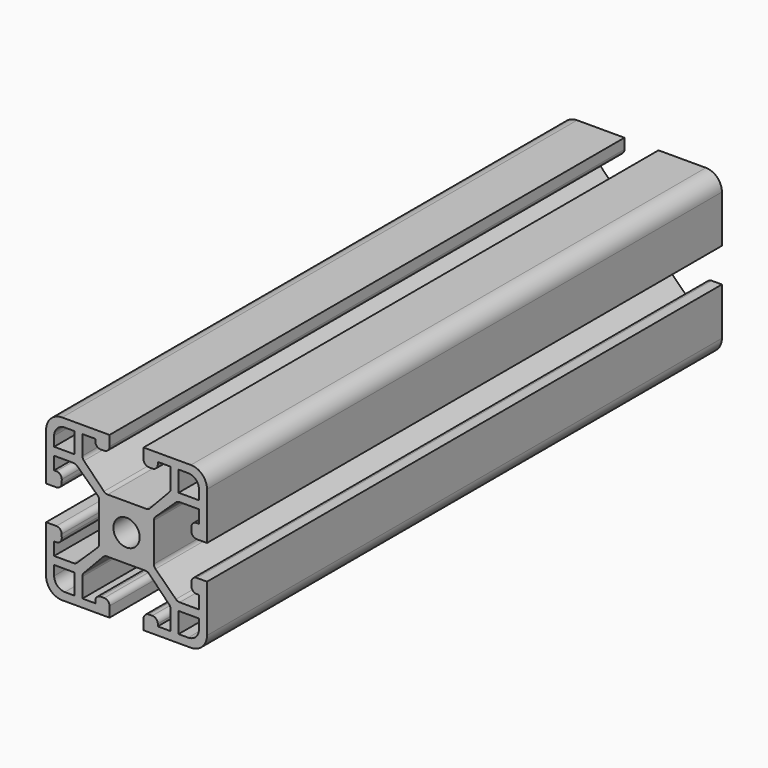
from build123d import *

# Parameters (mm, degrees)
F0_R     = 2.45
F1_DEPTH = 460
F2_DEPTH = 340


# Not quite as in the source:
# - ends of sketch curves that miss each other by under 0.0002 mm in the source are joined


with BuildPart() as f1:
    # F0 (on Front) → F1 (new body)
    with BuildSketch(Plane.XZ):
        with BuildLine():
            Line((-3.1749674082, 15), (-12, 15))
            ThreePointArc((-12, 15), (-14.1213203436, 14.1213203436), (-15, 12))
            Line((-15, 12), (-15, 3.175))
            Line((-15, 3.175), (-13.0855346263, 3.175))
            ThreePointArc((-13.0855346263, 3.175), (-12.3835980145, 3.4627605788), (-12.0856407741, 4.1604300138))
            Line((-12.0856407741, 4.1604300138), (-12.0761692778, 4.8104300138))
            ThreePointArc((-12.0761692778, 4.8104300138), (-12.3638237087, 5.5269366118), (-13.0760631299, 5.825))
            Line((-13.0760631299, 5.825), (-13.5, 5.825))
            Line((-13.5, 5.825), (-13.5, 8.225))
            Line((-13.5, 8.225), (-9.8968845016, 8.225))
            ThreePointArc((-9.8968845016, 8.225), (-9.5279915195, 8.1544718757), (-9.2111331975, 7.9528359354))
            Line((-9.2111331975, 7.9528359354), (-5.4142486959, 4.3754933338))
            ThreePointArc((-5.4142486959, 4.3754933338), (-5.1819174045, 4.0440465354), (-5.1, 3.6476573984))
            Line((-5.1, 3.6476573984), (-5.1, -3.4999243287))
            ThreePointArc((-5.1, -3.4999243287), (-5.1782354607, -3.8876744211), (-5.4007002683, -4.2147528992))
            Line((-5.4007002683, -4.2147528992), (-9.2084959767, -7.9398285705))
            ThreePointArc((-9.2084959767, -7.9398285705), (-9.5301904718, -8.1509666761), (-9.9077957084, -8.225))
            Line((-9.9077957084, -8.225), (-13.5, -8.225))
            Line((-13.5, -8.225), (-13.5, -5.825))
            Line((-13.5, -5.825), (-13.0760631299, -5.825))
            ThreePointArc((-13.0760631299, -5.825), (-12.3638237087, -5.5269366118), (-12.0761692778, -4.8104300138))
            Line((-12.0761692778, -4.8104300138), (-12.0856407741, -4.1604300138))
            ThreePointArc((-12.0856407741, -4.1604300138), (-12.3835980145, -3.4627605788), (-13.0855346263, -3.175))
            Line((-13.0855346263, -3.175), (-15, -3.175))
            Line((-15, -3.175), (-15, -12))
            ThreePointArc((-15, -12), (-14.1213203436, -14.1213203436), (-12, -15))
            Line((-12, -15), (-3.175, -15))
            Line((-3.175, -15), (-3.175, -13.0855346263))
            ThreePointArc((-3.175, -13.0855346263), (-3.4627605788, -12.3835980145), (-4.1604300138, -12.0856407741))
            Line((-4.1604300138, -12.0856407741), (-4.8104300138, -12.0761692778))
            ThreePointArc((-4.8104300138, -12.0761692778), (-5.5269366118, -12.3638237087), (-5.825, -13.0760631299))
            Line((-5.825, -13.0760631299), (-5.825, -13.5))
            Line((-5.825, -13.5), (-8.225, -13.5))
            Line((-8.225, -13.5), (-8.225, -9.8968845016))
            ThreePointArc((-8.225, -9.8968845016), (-8.1544718757, -9.5279915195), (-7.9528359354, -9.2111331975))
            Line((-7.9528359354, -9.2111331975), (-4.3754933338, -5.4142486959))
            ThreePointArc((-4.3754933338, -5.4142486959), (-4.0440465354, -5.1819174045), (-3.6476573984, -5.1))
            Line((-3.6476573984, -5.1), (3.4999243287, -5.1))
            ThreePointArc((3.4999243287, -5.1), (3.8876744211, -5.1782354607), (4.2147528992, -5.4007002683))
            Line((4.2147528992, -5.4007002683), (7.9398285705, -9.2084959767))
            ThreePointArc((7.9398285705, -9.2084959767), (8.1509666761, -9.5301904718), (8.225, -9.9077957084))
            Line((8.225, -9.9077957084), (8.225, -13.5))
            Line((8.225, -13.5), (5.825, -13.5))
            Line((5.825, -13.5), (5.825, -13.0760631299))
            ThreePointArc((5.825, -13.0760631299), (5.5269366118, -12.3638237087), (4.8104300138, -12.0761692778))
            Line((4.8104300138, -12.0761692778), (4.1604300138, -12.0856407741))
            ThreePointArc((4.1604300138, -12.0856407741), (3.4627605788, -12.3835980145), (3.175, -13.0855346263))
            Line((3.175, -13.0855346263), (3.175, -15))
            Line((3.175, -15), (12, -15))
            ThreePointArc((12, -15), (14.1213203436, -14.1213203436), (15, -12))
            Line((15, -12), (15, -3.175))
            Line((15, -3.175), (13.0855346263, -3.175))
            ThreePointArc((13.0855346263, -3.175), (12.3835980145, -3.4627605788), (12.0856407741, -4.1604300138))
            Line((12.0856407741, -4.1604300138), (12.0761692778, -4.8104300138))
            ThreePointArc((12.0761692778, -4.8104300138), (12.3638237087, -5.5269366118), (13.0760631299, -5.825))
            Line((13.0760631299, -5.825), (13.5, -5.825))
            Line((13.5, -5.825), (13.5, -8.225))
            Line((13.5, -8.225), (9.9077957084, -8.225))
            ThreePointArc((9.9077957084, -8.225), (9.5301904718, -8.1509666761), (9.2084959767, -7.9398285705))
            Line((9.2084959767, -7.9398285705), (5.4007002683, -4.2147528992))
            ThreePointArc((5.4007002683, -4.2147528992), (5.1782354607, -3.8876744211), (5.1, -3.4999243287))
            Line((5.1, -3.4999243287), (5.1, 3.6476573984))
            ThreePointArc((5.1, 3.6476573984), (5.1819174045, 4.0440465354), (5.4142486959, 4.3754933338))
            Line((5.4142486959, 4.3754933338), (9.2111331975, 7.9528359354))
            ThreePointArc((9.2111331975, 7.9528359354), (9.5279915195, 8.1544718757), (9.8968845016, 8.225))
            Line((9.8968845016, 8.225), (13.5, 8.225))
            Line((13.5, 8.225), (13.5, 5.825))
            Line((13.5, 5.825), (13.0760631299, 5.825))
            ThreePointArc((13.0760631299, 5.825), (12.3638237087, 5.5269366118), (12.0761692778, 4.8104300138))
            Line((12.0761692778, 4.8104300138), (12.0856407741, 4.1604300138))
            ThreePointArc((12.0856407741, 4.1604300138), (12.3835980145, 3.4627605788), (13.0855346263, 3.175))
            Line((13.0855346263, 3.175), (15, 3.175))
            Line((15, 3.175), (15, 12))
            ThreePointArc((15, 12), (14.1213203436, 14.1213203436), (12, 15))
            Line((12, 15), (3.1750325918, 15))
            Line((3.1750325918, 15), (3.1750325918, 13.0854824722))
            ThreePointArc((3.1750325918, 13.0854824722), (3.4627931706, 12.3835458604), (4.1604626057, 12.0855886201))
            Line((4.1604626057, 12.0855886201), (4.8104626057, 12.0761171237))
            ThreePointArc((4.8104626057, 12.0761171237), (5.5269692036, 12.3637715546), (5.8250325918, 13.0760109758))
            Line((5.8250325918, 13.0760109758), (5.8250325918, 13.4999478459))
            Line((5.8250325918, 13.4999478459), (8.2250325918, 13.4999478459))
            Line((8.2250325918, 13.4999478459), (8.2250325918, 9.8968323476))
            ThreePointArc((8.2250325918, 9.8968323476), (8.1545044675, 9.5279393654), (7.9528685272, 9.2110810434))
            Line((7.9528685272, 9.2110810434), (4.3755259256, 5.4141965418))
            ThreePointArc((4.3755259256, 5.4141965418), (4.0440791272, 5.1818652505), (3.6476899902, 5.0999478459))
            Line((3.6476899902, 5.0999478459), (-3.4998917369, 5.0999478459))
            ThreePointArc((-3.4998917369, 5.0999478459), (-3.8876418293, 5.1781833067), (-4.2147203074, 5.4006481142))
            Line((-4.2147203074, 5.4006481142), (-7.9397959787, 9.2084438226))
            ThreePointArc((-7.9397959787, 9.2084438226), (-8.1509340843, 9.5301383177), (-8.2249674082, 9.9077435543))
            Line((-8.2249674082, 9.9077435543), (-8.2249674082, 13.4999478459))
            Line((-8.2249674082, 13.4999478459), (-5.8249674082, 13.4999478459))
            Line((-5.8249674082, 13.4999478459), (-5.8249674082, 13.0760109758))
            ThreePointArc((-5.8249674082, 13.0760109758), (-5.5269040199, 12.3637715546), (-4.810397422, 12.0761171237))
            Line((-4.810397422, 12.0761171237), (-4.160397422, 12.0855886201))
            ThreePointArc((-4.160397422, 12.0855886201), (-3.462727987, 12.3835458604), (-3.1749674082, 13.0854824722))
            Line((-3.1749674082, 13.0854824722), (-3.1749674082, 15))
        make_face()
        with BuildLine():
            Line((-13.5, -11.5), (-13.5, -9.7))
            Line((-13.5, -9.7), (-9.7, -9.7))
            Line((-9.7, -9.7), (-9.7, -13.5))
            Line((-9.7, -13.5), (-11.5, -13.5))
            ThreePointArc((-11.5, -13.5), (-12.9142135624, -12.9142135624), (-13.5, -11.5))
        make_face(mode=Mode.SUBTRACT)
        with BuildLine():
            Line((9.7, -9.7), (13.5, -9.7))
            Line((13.5, -9.7), (13.5, -11.5))
            ThreePointArc((13.5, -11.5), (12.9142135624, -12.9142135624), (11.5, -13.5))
            Line((11.5, -13.5), (9.7, -13.5))
            Line((9.7, -13.5), (9.7, -9.7))
        make_face(mode=Mode.SUBTRACT)
        with BuildLine():
            ThreePointArc((-13.5, 11.5), (-12.9142135624, 12.9142135624), (-11.5, 13.5))
            Line((-11.5, 13.5), (-9.7, 13.5))
            Line((-9.7, 13.5), (-9.7, 9.7))
            Line((-9.7, 9.7), (-13.5, 9.7))
            Line((-13.5, 9.7), (-13.5, 11.5))
        make_face(mode=Mode.SUBTRACT)
        Circle(F0_R, mode=Mode.SUBTRACT)
        with BuildLine():
            Line((9.7, 13.5), (11.5, 13.5))
            ThreePointArc((11.5, 13.5), (12.9142135624, 12.9142135624), (13.5, 11.5))
            Line((13.5, 11.5), (13.5, 9.7))
            Line((13.5, 9.7), (9.7, 9.7))
            Line((9.7, 9.7), (9.7, 13.5))
        make_face(mode=Mode.SUBTRACT)
    extrude(amount=F1_DEPTH)

    # F2 (cut): a face of the model
    f2_faces = [f1.faces().sort_by_distance(p)[0] for p in [
        (5.2291627207, -460, 12.6659491494),
    ]]
    extrude(f2_faces, amount=-F2_DEPTH, mode=Mode.SUBTRACT)


solid = f1.part
